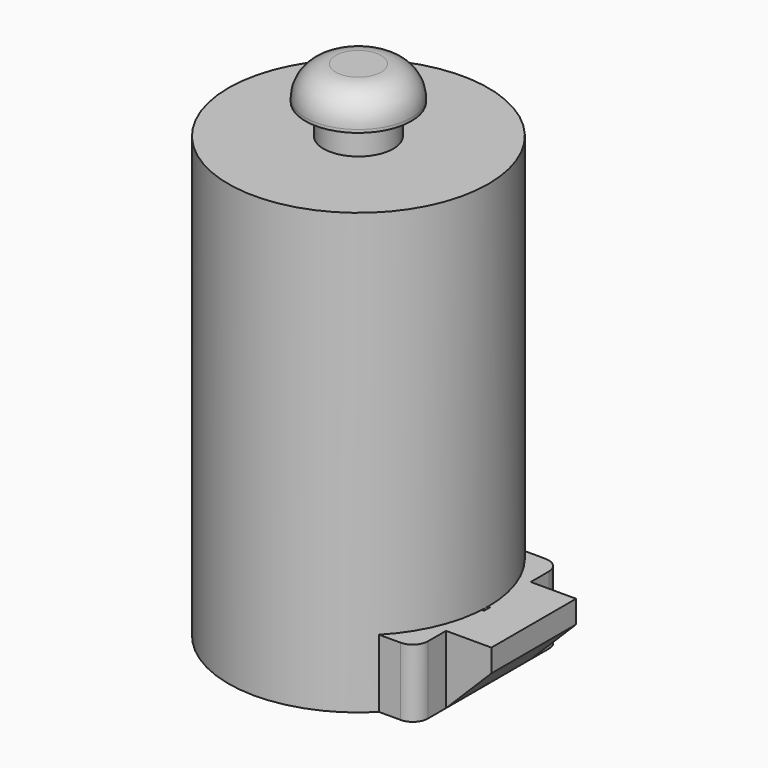
from build123d import *

# Parameters (mm, degrees)
F0_R         = 8.6
F0_R_2       = 7.25
F1_DEPTH     = 29.1
F2_R         = 8.6
F3_DEPTH     = 2.5
F4_R         = 3
F5_R         = 2.3
F6_DEPTH     = 2
F7_DEPTH     = 2
F8_R         = 3.5
F9_DEPTH     = 2.2
F10_R        = 2
F12_DEPTH    = 4.5
F13_T1_DEPTH = 22.4300979278
F14_R        = 1


# Not quite as in the source:
# - a fillet or chamfer that OpenCascade refuses, or shapes differently, is made with other operations: its cross-section is extruded or revolved along the edge and cut away or added


with BuildPart() as f1:
    # F0 (on Top) → F1 (new body)
    with BuildSketch(Plane.XY):
        Circle(F0_R)
        Circle(F0_R_2, mode=Mode.SUBTRACT)
    extrude(amount=F1_DEPTH)

    # F2 (on face) → F3 (join)
    with BuildSketch(Plane.XY.offset(29.1)):
        Circle(F2_R)
    extrude(amount=-F3_DEPTH)

    # F4
    f4_edges = [f1.edges().sort_by_distance(p)[0] for p in [
        (-7.25, 0, 26.6),
    ]]
    fillet(f4_edges, radius=F4_R)

    # F5 (on face) → F6 (join)
    with BuildSketch(Plane.XY.offset(29.1)):
        Circle(F5_R)
    extrude(amount=F6_DEPTH)

    # F5 (on face) → F7 (join)
    with BuildSketch(Plane.XY.offset(29.1)):
        Circle(F5_R)
    extrude(amount=-F7_DEPTH)

    # F8 (on face) → F9 (join)
    with BuildSketch(Plane.XY.offset(31.1)):
        Circle(F8_R)
    extrude(amount=F9_DEPTH)

    # F10
    f10_edges = [f1.edges().sort_by_distance(p)[0] for p in [
        (-3.5, 0, 33.3),
    ]]
    fillet(f10_edges, radius=F10_R)

    # F11 (on face) → F12 (join)
    with BuildSketch(Plane(origin=(0, 0, 0), x_dir=(1, 0, 0), z_dir=(0, 0, -1))):
        Polygon((8.6, -3.5), (8.6, 0), (7.3356842622, 0), (7.3356842622, -6), (8.6, -6), align=None)
        Polygon((7.3356842622, 0), (8.6, 0), (8.6, 0.5253988202), (8.6, 3.5), (8.6, 6), (7.3356842622, 6), align=None)
        Polygon((8.7317479774, 0), (8.6, 0), (8.6, -3.5), (11.6, -3.5), (11.6, 0), align=None)
        with BuildLine():
            Line((7.3356842622, -6), (7.3356842622, 0))
            Line((7.3356842622, 0), (7.3356842622, 6))
            Line((7.3356842622, 6), (6.1521958246, 6))
            Line((6.1521958246, 6), (6.1521958246, 3.8678361166))
            ThreePointArc((6.1521958246, 3.8678361166), (7.267026193, 0), (6.1521958246, -3.8678361166))
            Line((6.1521958246, -3.8678361166), (6.1521958246, -6.0092001577))
            Line((6.1521958246, -6.0092001577), (7.3356842622, -6.0092001577))
            Line((7.3356842622, -6.0092001577), (7.3356842622, -6))
        make_face()
        Polygon((8.6, 3.5), (8.6, 0.5253988202), (8.7317479774, 0.5253988202), (8.7317479774, 0), (11.6, 0), (11.6, 3.5), align=None)
    extrude(amount=-F12_DEPTH)

    # F13: chamfer of 3 on 1 edges, made by hand

    # F13_s2 → F13_t1 (cut)
    with BuildSketch(Plane.XZ.offset(-11.2150489639)):
        Polygon((8.6, 0), (11.6, 3), (11.6, 0), align=None)
    extrude(amount=F13_T1_DEPTH, mode=Mode.SUBTRACT)

    # F14
    f14_edges = [f1.edges().sort_by_distance(p)[0] for p in [
        (8.6, 6, 2.25),
        (8.6, -6, 2.25),
    ]]
    fillet(f14_edges, radius=F14_R)


solid = f1.part
